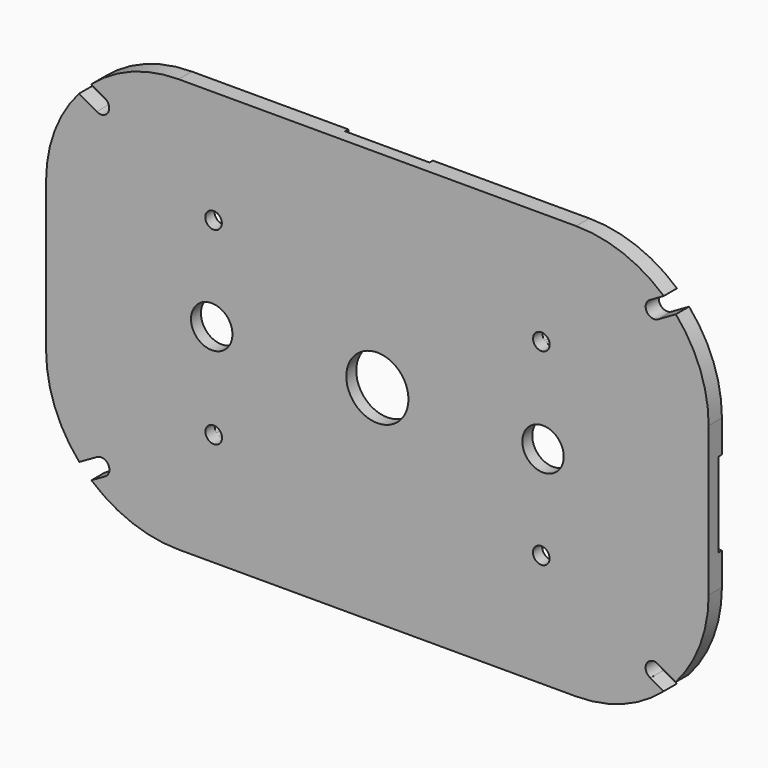
from build123d import *

# Parameters (mm, degrees)
F1_DEPTH  = 2.54
F3_DEPTH  = 12.7
F5_DEPTH  = 52.071
F7_DEPTH  = 76.2
F9_DEPTH  = 25.4
F10_W     = 50.673
F10_H     = 12.954
F10_W_2   = 12.954
F10_H_2   = 37.973
F11_DEPTH = 0.635
F12_DEPTH = 13.462
F14_DEPTH = 1.905
F15_R     = 4.7625
F15_R_2   = 3.175
F16_DEPTH = 25.4
F17_R     = 1.2763153823
F17_R_2   = 1.27
F18_DEPTH = 25.4


# Not quite as in the source:
# - ends of sketch curves that miss each other by under 0.0002 mm in the source are joined


with BuildPart() as f1:
    # F0 (on Front) → F1 (new body)
    with BuildSketch(Plane.XZ):
        with BuildLine():
            Line((30.48, 31.75), (-30.48, 31.75))
            ThreePointArc((-30.48, 31.75), (-44.8484097937, 25.7984097937), (-50.8, 11.43))
            Line((-50.8, 11.43), (-50.8, -11.43))
            ThreePointArc((-50.8, -11.43), (-44.8484097937, -25.7984097937), (-30.48, -31.75))
            Line((-30.48, -31.75), (30.48, -31.75))
            ThreePointArc((30.48, -31.75), (44.8484097937, -25.7984097937), (50.8, -11.43))
            Line((50.8, -11.43), (50.8, 11.43))
            ThreePointArc((50.8, 11.43), (44.8484097937, 25.7984097937), (30.48, 31.75))
        make_face()
    extrude(amount=F1_DEPTH)

    # F2 (on Front) → F3 (join)
    with BuildSketch(Plane.XZ):
        with BuildLine():
            ThreePointArc((33.02, 0), (27.0684097937, 14.3684097937), (12.7, 20.32))
            Line((12.7, 20.32), (-12.7, 20.32))
            ThreePointArc((-12.7, 20.32), (-27.0684097937, 14.3684097937), (-33.02, 0))
            ThreePointArc((-33.02, 0), (-27.0684097937, -14.3684097937), (-12.7, -20.32))
            Line((-12.7, -20.32), (12.7, -20.32))
            ThreePointArc((12.7, -20.32), (27.0684097937, -14.3684097937), (33.02, 0))
        make_face()
        with BuildLine():
            ThreePointArc((-30.48, 0), (-25.2723585695, 12.5723585695), (-12.7, 17.78))
            Line((-12.7, 17.78), (12.7, 17.78))
            ThreePointArc((12.7, 17.78), (25.2723585695, 12.5723585695), (30.48, 0))
            ThreePointArc((30.48, 0), (25.2723585695, -12.5723585695), (12.7, -17.78))
            Line((12.7, -17.78), (-12.7, -17.78))
            ThreePointArc((-12.7, -17.78), (-25.2723585695, -12.5723585695), (-30.48, 0))
        make_face(mode=Mode.SUBTRACT)
    extrude(amount=-F3_DEPTH)

    # F4 (on face) → F5 (cut, through all)
    with BuildSketch(Plane.XY.offset(20.32)):
        Polygon((6.604, 12.7), (0, 12.7), (-6.604, 12.7), (-6.604, 0), (6.604, 0), align=None)
    extrude(amount=-F5_DEPTH, mode=Mode.SUBTRACT)

    # F6 (on Right) → F7 (cut, symmetric)
    with BuildSketch(Plane.YZ):
        Polygon((0, 6.604), (0, 0), (0, -6.604), (12.7, -6.604), (12.7, 6.604), align=None)
    extrude(amount=F7_DEPTH, both=True, mode=Mode.SUBTRACT)

    # F8 (on face) → F9 (cut)
    with BuildSketch(Plane(origin=(0, 0, 0), x_dir=(-1, 0, 0), z_dir=(0, 1, 0))):
        with BuildLine():
            Line((12.7, 15.875), (-12.7, 15.875))
            ThreePointArc((-12.7, 15.875), (-23.9253201513, 11.2253201513), (-28.575, 0))
            ThreePointArc((-28.575, 0), (-23.9253201513, -11.2253201513), (-12.7, -15.875))
            Line((-12.7, -15.875), (12.7, -15.875))
            ThreePointArc((12.7, -15.875), (23.9253201513, -11.2253201513), (28.575, 0))
            ThreePointArc((28.575, 0), (23.9253201513, 11.2253201513), (12.7, 15.875))
        make_face()
    extrude(amount=-F9_DEPTH, mode=Mode.SUBTRACT)

    # F10 (on face) → F11 (cut)
    with BuildSketch(Plane(origin=(0, 0, 0), x_dir=(-1, 0, 0), z_dir=(0, 1, 0))):
        with Locations((-31.8135, 0)):
            Rectangle(F10_W, F10_H)
        with Locations((0, 25.4635)):
            Rectangle(F10_W_2, F10_H_2)
        Rectangle(F10_W_2, F10_H)
        with Locations((31.8135, 0)):
            Rectangle(F10_W, F10_H)
        with Locations((0, -25.4635)):
            Rectangle(F10_W_2, F10_H_2)
    extrude(amount=-F11_DEPTH, mode=Mode.SUBTRACT)

    # F12 (cut): faces of the model
    f12_faces = [f1.faces().sort_by_distance(p)[0] for p in [
        (9.652, 12.7, -20.0320986266),
        (30.5624774214, 12.7, 6.8919013734),
        (-30.5624774214, 12.7, -6.8919013734),
        (-6.8919013734, 12.7, 19.05),
    ]]
    extrude(f12_faces, amount=-F12_DEPTH, mode=Mode.SUBTRACT)

    # F13 (on face) → F14 (join)
    with BuildSketch(Plane.XZ.offset(2.54)):
        with BuildLine():
            Line((-12.7, -15.875), (12.7, -15.875))
            ThreePointArc((12.7, -15.875), (23.9253201513, -11.2253201513), (28.575, 0))
            ThreePointArc((28.575, 0), (23.9253201513, 11.2253201513), (12.7, 15.875))
            Line((12.7, 15.875), (-12.7, 15.875))
            ThreePointArc((-12.7, 15.875), (-23.9253201513, 11.2253201513), (-28.575, 0))
            ThreePointArc((-28.575, 0), (-23.9253201513, -11.2253201513), (-12.7, -15.875))
        make_face()
    extrude(amount=-F14_DEPTH)

    # F15 (on face) → F16 (cut)
    with BuildSketch(Plane(origin=(0, -0.635, 0), x_dir=(-1, 0, 0), z_dir=(0, 1, 0))):
        Circle(F15_R)
        with Locations((-25.4, 0)):
            Circle(F15_R_2)
        with Locations((25.4, 0)):
            Circle(F15_R_2)
    extrude(amount=-F16_DEPTH, mode=Mode.SUBTRACT)

    # F17 (on face) → F18 (cut)
    with BuildSketch(Plane(origin=(0, 0, 0), x_dir=(-1, 0, 0), z_dir=(0, 1, 0))):
        Polygon((47.6680542115, -27.4815886288), (51.1667876586, -29.4946501669), (47.6696745814, -27.4787697193), align=None)
        with BuildLine():
            Line((47.0404791933, -28.5733623005), (47.6680542115, -27.4815886288))
            Line((47.6680542115, -27.4815886288), (47.6696745814, -27.4787697193))
            Line((47.6696745814, -27.4787697193), (48.3063004883, -26.3712504847))
            Line((48.3063004883, -26.3712504847), (43.0570225864, -23.3538525016))
            ThreePointArc((43.0570225864, -23.3538525016), (41.2580877478, -23.7846525937), (41.7912012914, -25.5559643173))
            Line((41.7912012914, -25.5559643173), (47.0404791933, -28.5733623005))
        make_face()
        with Locations((-25.1277598759, -14.4543864422)):
            Circle(F17_R)
        with Locations((-25.1438466209, 14.4120964147)):
            Circle(F17_R_2)
        with Locations((25.1215984181, 14.4508421512)):
            Circle(F17_R_2)
        with Locations((25.0963969645, -14.4945646834)):
            Circle(F17_R_2)
        with BuildLine():
            ThreePointArc((-41.8649914427, -25.5417502167), (-41.2719571065, -23.8052669732), (-43.0327445767, -23.2888453782))
            Line((-43.0327445767, -23.2888453782), (-48.1358024341, -26.2243068229))
            Line((-48.1358024341, -26.2243068229), (-46.8692956724, -28.4260244757))
            Line((-46.8692956724, -28.4260244757), (-41.8629335005, -25.5461858486))
            Line((-41.8629335005, -25.5461858486), (-41.8649914427, -25.5417502167))
        make_face()
        with BuildLine():
            ThreePointArc((-43.0465700311, 23.2475518967), (-41.3065716807, 23.7045275153), (-41.7691664779, 25.443040394))
            Line((-41.7691664779, 25.443040394), (-41.7793320219, 25.4488488271))
            Line((-41.7793320219, 25.4488488271), (-42.2095022754, 25.6963553049))
            Line((-42.2095022754, 25.6963553049), (-46.0359033246, 27.8979465087))
            Line((-46.0359033246, 27.8979465087), (-47.302629882, 25.6963553049))
            Line((-47.302629882, 25.6963553049), (-43.0465700311, 23.2475518967))
        make_face()
        with BuildLine():
            Line((46.6254135383, 28.2857347472), (41.7498114349, 25.4811139895))
            ThreePointArc((41.7498114349, 25.4811139895), (41.2839564144, 23.7439684966), (43.0223799296, 23.2829055446))
            Line((43.0223799296, 23.2829055446), (47.8919203, 26.0840170944))
            Line((47.8919203, 26.0840170944), (46.6254135383, 28.2857347472))
        make_face()
    extrude(amount=-F18_DEPTH, mode=Mode.SUBTRACT)


solid = f1.part
